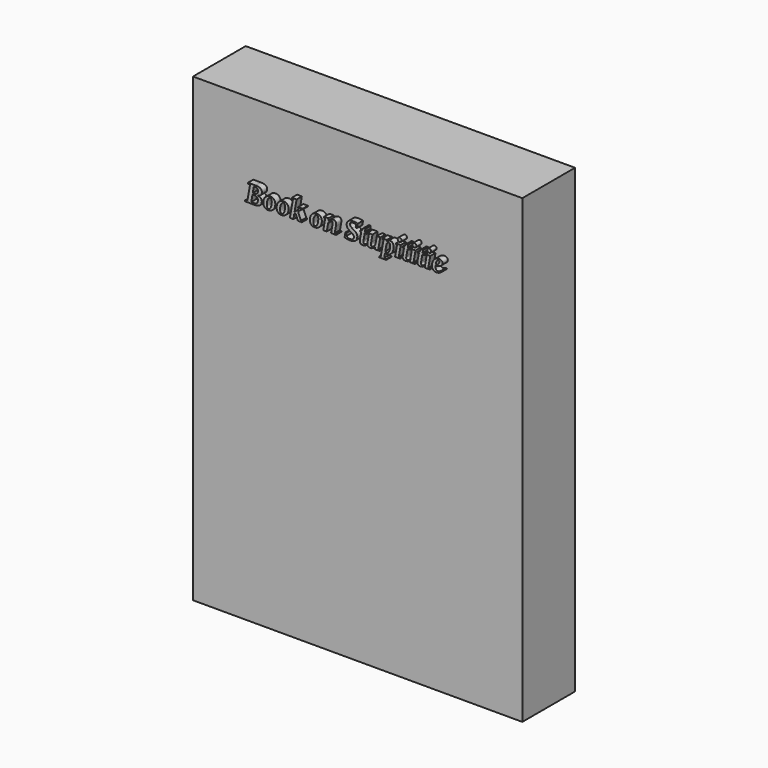
from build123d import *

# Parameters (mm, degrees)
F0_W         = 127
F0_H         = 177.8
F1_DEPTH     = 25.4
F3_TEXT_SIZE = 10.2511929035
F4_DEPTH     = 2.54


# Not quite as in the source:
# - Text() gives the source's letters only with a copy of the font that has no kerning and outlines rounded to 1/6400 em; it was checked with that copy


with BuildPart() as f1:
    # F0 (on Front) → F1 (new body)
    with BuildSketch(Plane.XZ):
        Rectangle(F0_W, F0_H)
    extrude(amount=F1_DEPTH)

    # F3 (on face) → F4 (join)
    with BuildSketch(Plane.XZ.offset(25.4)):
        with Locations((-41.3407044765, 54.7406927533)):
            Text('Book on Stupititie', F3_TEXT_SIZE, font='Tinos', font_style=FontStyle.BOLDITALIC, text_align=(TextAlign.LEFT, TextAlign.BOTTOM))
    extrude(amount=F4_DEPTH)


solid = f1.part
